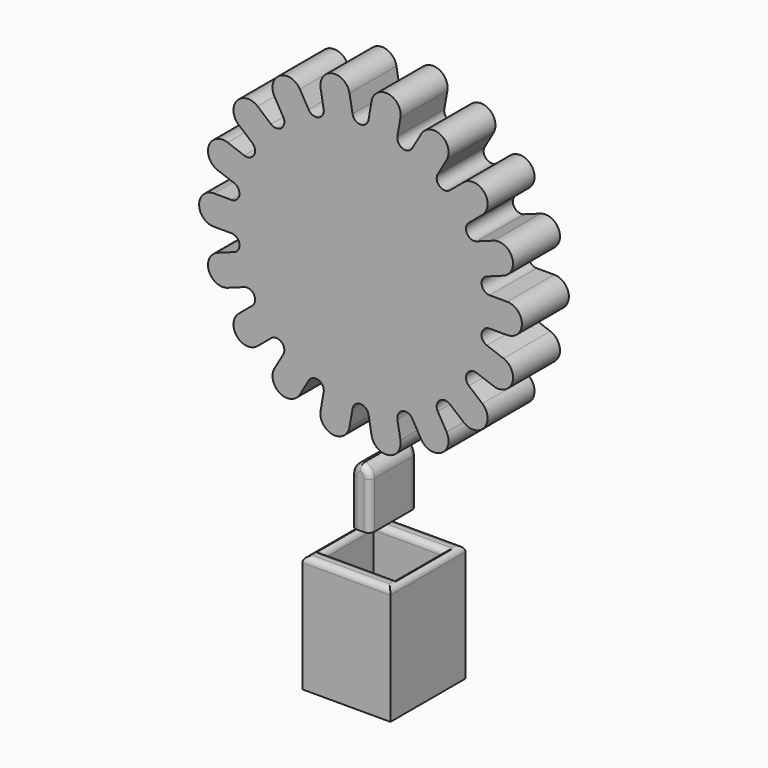
from build123d import *

# Parameters (mm, degrees)
F1_DEPTH      = 5
F1_DEPTH_BACK = 5
F2_W          = 3.2
F2_H          = 10
F3_DEPTH      = 5
F3_DEPTH_BACK = 5
F4_T1_DEPTH   = 20
F5_T1_DEPTH   = 10.5
F5_T4_ANGLE   = 150.1046308582
F5_T6_ANGLE   = 150.1046308582
F5_T8_ANGLE   = 150.1046308582
F5_T10_ANGLE  = 150.1046308582
F6_W          = 15
F6_H          = 20
F7_DEPTH      = 8
F7_DEPTH_BACK = 8
F8_W          = 12
F8_H          = 10.5
F9_DEPTH      = 10
F10_T1_DEPTH  = 21
F10_T3_DEPTH  = 20
F10_T5_DEPTH  = 10.5
F10_T7_DEPTH  = 12
F10_T13_DEPTH = 13
F10_T17_DEPTH = 14.5
F10_T24_DEPTH = 13
F10_T28_DEPTH = 14.5
F10_T35_DEPTH = 14.5
F10_T39_DEPTH = 13
F10_T46_DEPTH = 13
F10_T50_DEPTH = 14.5


# Not quite as in the source:
# - a fillet or chamfer that OpenCascade refuses, or shapes differently, is made with other operations: its cross-section is extruded or revolved along the edge and cut away or added


with BuildPart() as f1:
    # F0 (on Front) → F1 (new body, two sides)
    with BuildSketch(Plane.XZ) as f1_sk:
        with BuildLine():
            ThreePointArc((-21.5282880156, 5.1752116012), (-20.6417594739, 3.6396991245), (-22, 2.5))
            Line((-22, 2.5), (-25, 2.5))
            ThreePointArc((-25, 2.5), (-27.5, 0), (-25, -2.5))
            Line((-25, -2.5), (-22, -2.5))
            ThreePointArc((-22, -2.5), (-20.6417594739, -3.6396991245), (-21.5282880156, -5.1752116012))
            Line((-21.5282880156, -5.1752116012), (-24.347365878, -6.2012720312))
            ThreePointArc((-24.347365878, -6.2012720312), (-25.8415470716, -9.4055539415), (-22.6372651613, -10.8997351351))
            Line((-22.6372651613, -10.8997351351), (-19.818187299, -9.8736747051))
            ThreePointArc((-19.818187299, -9.8736747051), (-18.1520586414, -10.480095943), (-18.4599467728, -12.2262163053))
            Line((-18.4599467728, -12.2262163053), (-20.7580801022, -14.1545791344))
            ThreePointArc((-20.7580801022, -14.1545791344), (-21.0662221858, -17.6766592664), (-17.5441420538, -17.98480135))
            Line((-17.5441420538, -17.98480135), (-15.2460087244, -16.0564385209))
            ThreePointArc((-15.2460087244, -16.0564385209), (-13.4729516409, -16.0564385209), (-13.1650635095, -17.8025588833))
            Line((-13.1650635095, -17.8025588833), (-14.6650635095, -20.4006350946))
            ThreePointArc((-14.6650635095, -20.4006350946), (-13.75, -23.8156986041), (-10.3349364905, -22.9006350946))
            Line((-10.3349364905, -22.9006350946), (-8.8349364905, -20.3025588833))
            ThreePointArc((-8.8349364905, -20.3025588833), (-7.1688078329, -19.6961376454), (-6.2822792912, -21.2316501221))
            Line((-6.2822792912, -21.2316501221), (-6.8032238242, -24.1860733811))
            ThreePointArc((-6.8032238242, -24.1860733811), (-4.7753248858, -27.0822132078), (-1.8791850591, -25.0543142695))
            Line((-1.8791850591, -25.0543142695), (-1.3582405261, -22.0998910104))
            ThreePointArc((-1.3582405261, -22.0998910104), (0, -20.9601918859), (1.3582405261, -22.0998910104))
            Line((1.3582405261, -22.0998910104), (1.8791850591, -25.0543142695))
            ThreePointArc((1.8791850591, -25.0543142695), (4.7753248858, -27.0822132078), (6.8032238242, -24.1860733811))
            Line((6.8032238242, -24.1860733811), (6.2822792912, -21.2316501221))
            ThreePointArc((6.2822792912, -21.2316501221), (7.1688078329, -19.6961376454), (8.8349364905, -20.3025588833))
            Line((8.8349364905, -20.3025588833), (10.3349364905, -22.9006350946))
            ThreePointArc((10.3349364905, -22.9006350946), (13.75, -23.8156986041), (14.6650635095, -20.4006350946))
            Line((14.6650635095, -20.4006350946), (13.1650635095, -17.8025588833))
            ThreePointArc((13.1650635095, -17.8025588833), (13.4729516409, -16.0564385209), (15.2460087244, -16.0564385209))
            Line((15.2460087244, -16.0564385209), (17.5441420538, -17.98480135))
            ThreePointArc((17.5441420538, -17.98480135), (21.0662221858, -17.6766592664), (20.7580801022, -14.1545791344))
            Line((20.7580801022, -14.1545791344), (18.4599467728, -12.2262163053))
            ThreePointArc((18.4599467728, -12.2262163053), (18.1520586414, -10.480095943), (19.818187299, -9.8736747051))
            Line((19.818187299, -9.8736747051), (22.6372651613, -10.8997351351))
            ThreePointArc((22.6372651613, -10.8997351351), (25.8415470716, -9.4055539415), (24.347365878, -6.2012720312))
            Line((24.347365878, -6.2012720312), (21.5282880156, -5.1752116012))
            ThreePointArc((21.5282880156, -5.1752116012), (20.6417594739, -3.6396991245), (22, -2.5))
            Line((22, -2.5), (25, -2.5))
            ThreePointArc((25, -2.5), (27.5, 0), (25, 2.5))
            Line((25, 2.5), (22, 2.5))
            ThreePointArc((22, 2.5), (20.6417594739, 3.6396991245), (21.5282880156, 5.1752116012))
            Line((21.5282880156, 5.1752116012), (24.347365878, 6.2012720312))
            ThreePointArc((24.347365878, 6.2012720312), (25.8415470716, 9.4055539415), (22.6372651613, 10.8997351351))
            Line((22.6372651613, 10.8997351351), (19.818187299, 9.8736747051))
            ThreePointArc((19.818187299, 9.8736747051), (18.1520586414, 10.480095943), (18.4599467728, 12.2262163053))
            Line((18.4599467728, 12.2262163053), (20.7580801022, 14.1545791344))
            ThreePointArc((20.7580801022, 14.1545791344), (21.0662221858, 17.6766592664), (17.5441420538, 17.98480135))
            Line((17.5441420538, 17.98480135), (15.2460087244, 16.0564385209))
            ThreePointArc((15.2460087244, 16.0564385209), (13.4729516409, 16.0564385209), (13.1650635095, 17.8025588833))
            Line((13.1650635095, 17.8025588833), (14.6650635095, 20.4006350946))
            ThreePointArc((14.6650635095, 20.4006350946), (13.75, 23.8156986041), (10.3349364905, 22.9006350946))
            Line((10.3349364905, 22.9006350946), (8.8349364905, 20.3025588833))
            ThreePointArc((8.8349364905, 20.3025588833), (7.1688078329, 19.6961376454), (6.2822792912, 21.2316501221))
            Line((6.2822792912, 21.2316501221), (6.8032238242, 24.1860733811))
            ThreePointArc((6.8032238242, 24.1860733811), (4.7753248858, 27.0822132078), (1.8791850591, 25.0543142695))
            Line((1.8791850591, 25.0543142695), (1.3582405261, 22.0998910104))
            ThreePointArc((1.3582405261, 22.0998910104), (0, 20.9601918859), (-1.3582405261, 22.0998910104))
            Line((-1.3582405261, 22.0998910104), (-1.8791850591, 25.0543142695))
            ThreePointArc((-1.8791850591, 25.0543142695), (-4.7753248858, 27.0822132078), (-6.8032238242, 24.1860733811))
            Line((-6.8032238242, 24.1860733811), (-6.2822792912, 21.2316501221))
            ThreePointArc((-6.2822792912, 21.2316501221), (-7.1688078329, 19.6961376454), (-8.8349364905, 20.3025588833))
            Line((-8.8349364905, 20.3025588833), (-10.3349364905, 22.9006350946))
            ThreePointArc((-10.3349364905, 22.9006350946), (-13.75, 23.8156986041), (-14.6650635095, 20.4006350946))
            Line((-14.6650635095, 20.4006350946), (-13.1650635095, 17.8025588833))
            ThreePointArc((-13.1650635095, 17.8025588833), (-13.4729516409, 16.0564385209), (-15.2460087244, 16.0564385209))
            Line((-15.2460087244, 16.0564385209), (-17.5441420538, 17.98480135))
            ThreePointArc((-17.5441420538, 17.98480135), (-21.0662221858, 17.6766592664), (-20.7580801022, 14.1545791344))
            Line((-20.7580801022, 14.1545791344), (-18.4599467728, 12.2262163053))
            ThreePointArc((-18.4599467728, 12.2262163053), (-18.1520586414, 10.480095943), (-19.818187299, 9.8736747051))
            Line((-19.818187299, 9.8736747051), (-22.6372651613, 10.8997351351))
            ThreePointArc((-22.6372651613, 10.8997351351), (-25.8415470716, 9.4055539415), (-24.347365878, 6.2012720312))
            Line((-24.347365878, 6.2012720312), (-21.5282880156, 5.1752116012))
        make_face()
    extrude(amount=F1_DEPTH)
    extrude(f1_sk.sketch, amount=-F1_DEPTH_BACK)


with BuildPart() as f3:
    # F2 (on Front) → F3 (new body, two sides)
    with BuildSketch(Plane.XZ) as f3_sk:
        with Locations((0, -35)):
            Rectangle(F2_W, F2_H)
    extrude(amount=F3_DEPTH)
    extrude(f3_sk.sketch, amount=-F3_DEPTH_BACK)

    # F4: fillet of radius 2 on 2 edges, made by hand

    # F4_s2 → F4_t1 (cut)
    with BuildSketch(Plane.XZ.offset(-10)):
        with BuildLine():
            ThreePointArc((-1.6, -32), (-1.0142135624, -30.5857864376), (0.4, -30))
            Line((0.4, -30), (-1.6, -30))
            Line((-1.6, -30), (-1.6, -32))
        make_face()
        with BuildLine():
            ThreePointArc((1.6, -32), (1.0142135624, -30.5857864376), (-0.4, -30))
            Line((-0.4, -30), (1.6, -30))
            Line((1.6, -30), (1.6, -32))
        make_face()
    extrude(amount=F4_T1_DEPTH, mode=Mode.SUBTRACT)

    # F5: fillet of radius 1 on 4 edges, made by hand

    # F5_s2 → F5_t1 (cut)
    with BuildSketch(Plane.XY.offset(-42.5)):
        with BuildLine():
            ThreePointArc((-1.6, 4), (-1.3071067812, 4.7071067812), (-0.6, 5))
            Line((-0.6, 5), (-1.6, 5))
            Line((-1.6, 5), (-1.6, 4))
        make_face()
        with BuildLine():
            ThreePointArc((0.6, 5), (1.3071067812, 4.7071067812), (1.6, 4))
            Line((1.6, 4), (1.6, 5))
            Line((1.6, 5), (0.6, 5))
        make_face()
        with BuildLine():
            ThreePointArc((-1.6, -4), (-1.3071067812, -4.7071067812), (-0.6, -5))
            Line((-0.6, -5), (-1.6, -5))
            Line((-1.6, -5), (-1.6, -4))
        make_face()
        with BuildLine():
            ThreePointArc((0.6, -5), (1.3071067812, -4.7071067812), (1.6, -4))
            Line((1.6, -4), (1.6, -5))
            Line((1.6, -5), (0.6, -5))
        make_face()
    extrude(amount=F5_T1_DEPTH, mode=Mode.SUBTRACT)

    # F5_s3 → F5_t4 (revolve, cut)
    with BuildSketch(Plane(origin=(-13.9264637315, 0, -24.2233930604), x_dir=(0, 1, 0), z_dir=(-0.4984176723, 0, -0.8669370357))):
        with BuildLine():
            ThreePointArc((-5, 14.6025907008), (-4.7071067812, 13.8954839196), (-4, 13.6025907008))
            Line((-4, 13.6025907008), (-5, 13.6025907008))
            Line((-5, 13.6025907008), (-5, 14.6025907008))
        make_face()
    revolve(axis=Axis((-0.3999999999, -5, -31.9999999999), (0, 1, 0)), revolution_arc=F5_T4_ANGLE, mode=Mode.SUBTRACT)

    # F5_s5 → F5_t6 (revolve, cut)
    with BuildSketch(Plane.XY.offset(-31.9999999999)):
        with BuildLine():
            ThreePointArc((-1.6, -4), (-1.3071067812, -4.7071067812), (-0.6, -5))
            Line((-0.6, -5), (-1.6, -5))
            Line((-1.6, -5), (-1.6, -4))
        make_face()
    revolve(axis=Axis((0.3999999999, -5, -31.9999999999), (0, 1, 0)), revolution_arc=F5_T6_ANGLE, mode=Mode.SUBTRACT)

    # F5_s7 → F5_t8 (revolve, cut)
    with BuildSketch(Plane(origin=(-13.9264637315, 0, -24.2233930604), x_dir=(0, 1, 0), z_dir=(-0.4984176723, 0, -0.8669370357))):
        with BuildLine():
            ThreePointArc((5, 14.6025907008), (4.7071067812, 13.8954839196), (4, 13.6025907008))
            Line((4, 13.6025907008), (5, 13.6025907008))
            Line((5, 13.6025907008), (5, 14.6025907008))
        make_face()
    revolve(axis=Axis((-0.3999999999, 5, -31.9999999999), (0, 1, 0)), revolution_arc=F5_T8_ANGLE, mode=Mode.SUBTRACT)

    # F5_s9 → F5_t10 (revolve, cut)
    with BuildSketch(Plane.XY.offset(-31.9999999999)):
        with BuildLine():
            ThreePointArc((-1.6, 4), (-1.3071067812, 4.7071067812), (-0.6, 5))
            Line((-0.6, 5), (-1.6, 5))
            Line((-1.6, 5), (-1.6, 4))
        make_face()
    revolve(axis=Axis((0.3999999999, 5, -31.9999999999), (0, 1, 0)), revolution_arc=F5_T10_ANGLE, mode=Mode.SUBTRACT)


with BuildPart() as f7:
    # F6 (on Front) → F7 (new body, two sides)
    with BuildSketch(Plane.XZ) as f7_sk:
        with Locations((0, -55)):
            Rectangle(F6_W, F6_H)
    extrude(amount=F7_DEPTH)
    extrude(f7_sk.sketch, amount=-F7_DEPTH_BACK)

    # F8 (on face) → F9 (cut)
    with BuildSketch(Plane.XY.offset(-45)):
        Rectangle(F8_W, F8_H)
    extrude(amount=-F9_DEPTH, mode=Mode.SUBTRACT)

    # F10: fillet of radius 1 on 8 edges, made by hand

    # F10_s2 → F10_t1 (cut)
    with BuildSketch(Plane.XZ.offset(-10.5)):
        with BuildLine():
            ThreePointArc((6.5, -45), (7.2071067812, -45.2928932188), (7.5, -46))
            Line((7.5, -46), (7.5, -45))
            Line((7.5, -45), (6.5, -45))
        make_face()
        with BuildLine():
            ThreePointArc((-6.5, -45), (-7.2071067812, -45.2928932188), (-7.5, -46))
            Line((-7.5, -46), (-7.5, -45))
            Line((-7.5, -45), (-6.5, -45))
        make_face()
    extrude(amount=F10_T1_DEPTH, mode=Mode.SUBTRACT)

    # F10_s4 → F10_t3 (cut)
    with BuildSketch(Plane.YZ.offset(-10)):
        with BuildLine():
            ThreePointArc((-7, -45), (-7.7071067812, -45.2928932188), (-8, -46))
            Line((-8, -46), (-8, -45))
            Line((-8, -45), (-7, -45))
        make_face()
        with BuildLine():
            ThreePointArc((7, -45), (7.7071067812, -45.2928932188), (8, -46))
            Line((8, -46), (8, -45))
            Line((8, -45), (7, -45))
        make_face()
    extrude(amount=F10_T3_DEPTH, mode=Mode.SUBTRACT)

    # F10_s6 → F10_t5 (cut)
    with BuildSketch(Plane.XZ.offset(-5.25)):
        with BuildLine():
            ThreePointArc((7, -45), (6.2928932188, -45.2928932188), (6, -46))
            Line((6, -46), (6, -45))
            Line((6, -45), (7, -45))
        make_face()
        with BuildLine():
            ThreePointArc((-7, -45), (-6.2928932188, -45.2928932188), (-6, -46))
            Line((-6, -46), (-6, -45))
            Line((-6, -45), (-7, -45))
        make_face()
    extrude(amount=F10_T5_DEPTH, mode=Mode.SUBTRACT)

    # F10_s8 → F10_t7 (cut)
    with BuildSketch(Plane.YZ.offset(-6)):
        with BuildLine():
            ThreePointArc((-6.25, -45), (-5.5428932188, -45.2928932188), (-5.25, -46))
            Line((-5.25, -46), (-5.25, -45))
            Line((-5.25, -45), (-6.25, -45))
        make_face()
        with BuildLine():
            ThreePointArc((6.25, -45), (5.5428932188, -45.2928932188), (5.25, -46))
            Line((5.25, -46), (5.25, -45))
            Line((5.25, -45), (6.25, -45))
        make_face()
    extrude(amount=F10_T7_DEPTH, mode=Mode.SUBTRACT)


with BuildPart() as f10_tool11:
    # F10_s12 → F10_t13 (new body)
    with BuildSketch(Plane.XZ.offset(7.75)):
        with BuildLine():
            ThreePointArc((7, -45), (6.2928932188, -45.2928932188), (6, -46))
            Line((6, -46), (6, -45))
            Line((6, -45), (7, -45))
        make_face()
    extrude(amount=-F10_T13_DEPTH)

    split(bisect_by=Plane.XZ.offset(5.25), keep=Keep.TOP)


with BuildPart() as f10_tool15:
    # F10_s16 → F10_t17 (new body)
    with BuildSketch(Plane.YZ.offset(-6)):
        with BuildLine():
            ThreePointArc((-6.25, -45), (-5.5428932188, -45.2928932188), (-5.25, -46))
            Line((-5.25, -46), (-5.25, -45))
            Line((-5.25, -45), (-6.25, -45))
        make_face()
    extrude(amount=F10_T17_DEPTH)

    split(bisect_by=Plane.YZ.offset(6), keep=Keep.TOP)


with BuildPart() as f10_tool11_1:
    add(f10_tool11.part)

    # F10_t19: intersect F10_tool15
    add(f10_tool15.part, mode=Mode.INTERSECT)


with BuildPart() as f7_1:
    add(f7.part)

    # F10_t9: cut F10_tool11
    add(f10_tool11_1.part, mode=Mode.SUBTRACT)


with BuildPart() as f10_tool22:
    # F10_s23 → F10_t24 (new body)
    with BuildSketch(Plane.XZ.offset(5.25)):
        with BuildLine():
            ThreePointArc((7, -45), (6.2928932188, -45.2928932188), (6, -46))
            Line((6, -46), (6, -45))
            Line((6, -45), (7, -45))
        make_face()
    extrude(amount=-F10_T24_DEPTH)

    split(bisect_by=Plane.XZ.offset(-5.25), keep=Keep.BOTTOM)


with BuildPart() as f10_tool26:
    # F10_s27 → F10_t28 (new body)
    with BuildSketch(Plane.YZ.offset(8.5)):
        with BuildLine():
            ThreePointArc((6.25, -45), (5.5428932188, -45.2928932188), (5.25, -46))
            Line((5.25, -46), (5.25, -45))
            Line((5.25, -45), (6.25, -45))
        make_face()
    extrude(amount=-F10_T28_DEPTH)

    split(bisect_by=Plane.YZ.offset(6), keep=Keep.TOP)


with BuildPart() as f10_tool22_1:
    add(f10_tool22.part)

    # F10_t30: intersect F10_tool26
    add(f10_tool26.part, mode=Mode.INTERSECT)


with BuildPart() as f7_2:
    add(f7_1.part)

    # F10_t20: cut F10_tool22
    add(f10_tool22_1.part, mode=Mode.SUBTRACT)


with BuildPart() as f10_tool33:
    # F10_s34 → F10_t35 (new body)
    with BuildSketch(Plane.YZ.offset(-8.5)):
        with BuildLine():
            ThreePointArc((-6.25, -45), (-5.5428932188, -45.2928932188), (-5.25, -46))
            Line((-5.25, -46), (-5.25, -45))
            Line((-5.25, -45), (-6.25, -45))
        make_face()
    extrude(amount=F10_T35_DEPTH)

    split(bisect_by=Plane.YZ.offset(-6), keep=Keep.BOTTOM)


with BuildPart() as f10_tool37:
    # F10_s38 → F10_t39 (new body)
    with BuildSketch(Plane.XZ.offset(-5.25)):
        with BuildLine():
            ThreePointArc((-7, -45), (-6.2928932188, -45.2928932188), (-6, -46))
            Line((-6, -46), (-6, -45))
            Line((-6, -45), (-7, -45))
        make_face()
    extrude(amount=F10_T39_DEPTH)

    split(bisect_by=Plane.XZ.offset(5.25), keep=Keep.TOP)


with BuildPart() as f10_tool33_1:
    add(f10_tool33.part)

    # F10_t41: intersect F10_tool37
    add(f10_tool37.part, mode=Mode.INTERSECT)


with BuildPart() as f7_3:
    add(f7_2.part)

    # F10_t31: cut F10_tool33
    add(f10_tool33_1.part, mode=Mode.SUBTRACT)


with BuildPart() as f10_tool44:
    # F10_s45 → F10_t46 (new body)
    with BuildSketch(Plane.XZ.offset(-7.75)):
        with BuildLine():
            ThreePointArc((-7, -45), (-6.2928932188, -45.2928932188), (-6, -46))
            Line((-6, -46), (-6, -45))
            Line((-6, -45), (-7, -45))
        make_face()
    extrude(amount=F10_T46_DEPTH)

    split(bisect_by=Plane.XZ.offset(-5.25), keep=Keep.BOTTOM)


with BuildPart() as f10_tool48:
    # F10_s49 → F10_t50 (new body)
    with BuildSketch(Plane.YZ.offset(6)):
        with BuildLine():
            ThreePointArc((6.25, -45), (5.5428932188, -45.2928932188), (5.25, -46))
            Line((5.25, -46), (5.25, -45))
            Line((5.25, -45), (6.25, -45))
        make_face()
    extrude(amount=-F10_T50_DEPTH)

    split(bisect_by=Plane.YZ.offset(-6), keep=Keep.BOTTOM)


with BuildPart() as f10_tool44_1:
    add(f10_tool44.part)

    # F10_t52: intersect F10_tool48
    add(f10_tool48.part, mode=Mode.INTERSECT)


with BuildPart() as f7_4:
    add(f7_3.part)

    # F10_t42: cut F10_tool44
    add(f10_tool44_1.part, mode=Mode.SUBTRACT)


solid = Compound([f1.part, f3.part, f7_4.part])
